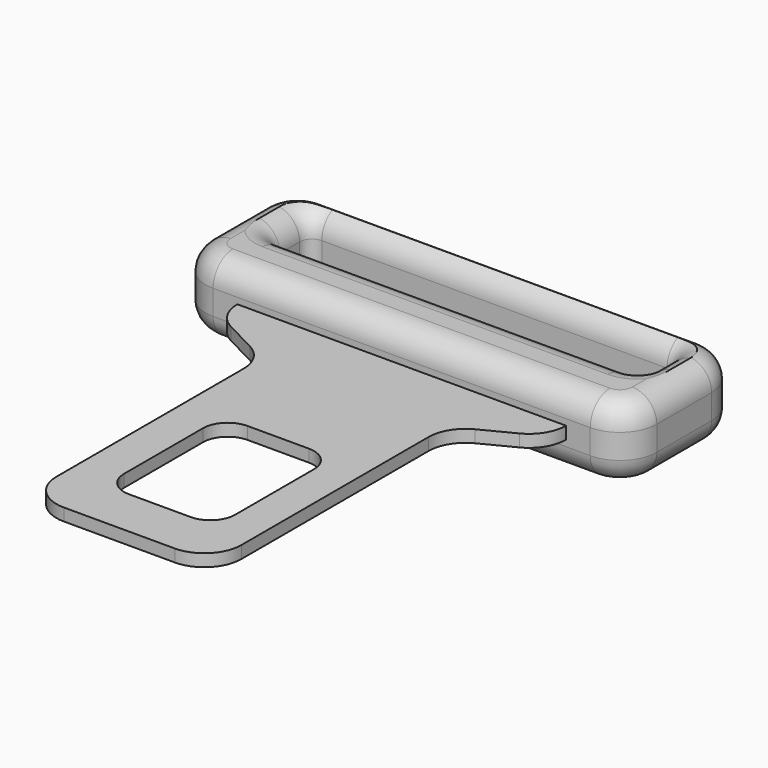
from build123d import *

# Parameters (mm, degrees)
F1_DEPTH     = 0.5
F2_DEPTH     = 3
F3_T1_DEPTH  = 30.5823954344
F3_T3_DEPTH  = 28
F3_T5_DEPTH  = 2
F3_T7_DEPTH  = 5.5512716671
F3_T10_ANGLE = 90
F3_T12_ANGLE = 90
F3_T14_ANGLE = 90
F3_T16_ANGLE = 90
F3_T18_ANGLE = 90
F3_T20_ANGLE = 90
F3_T22_ANGLE = 90
F3_T24_ANGLE = 90
F3_T26_ANGLE = 90
F3_T28_ANGLE = 90
F3_T30_ANGLE = 90
F3_T32_ANGLE = 90
F3_T34_ANGLE = 90
F3_T36_ANGLE = 90
F3_T38_ANGLE = 90
F3_T40_ANGLE = 90


# Not quite as in the source:
# - a fillet or chamfer that OpenCascade refuses, or shapes differently, is made with other operations: its cross-section is extruded or revolved along the edge and cut away or added
# - ends of sketch curves that miss each other by under 0.0002 mm in the source are joined


with BuildPart() as f1:
    # F0 (on Top) → F1 (new body, symmetric)
    with BuildSketch(Plane.XY):
        with BuildLine():
            ThreePointArc((-7.5000009313, -20.8021384721), (-6.6213212749, -22.9234588157), (-4.5000009313, -23.8021384721))
            Line((-4.5000009313, -23.8021384721), (4.4999990687, -23.8021384721))
            ThreePointArc((4.4999990687, -23.8021384721), (6.6213194122, -22.9234588157), (7.4999990687, -20.8021384721))
            Line((7.4999990687, -20.8021384721), (7.4999990687, -3.8021384721))
            Line((7.4999990687, -3.8021384721), (7.4999990687, -1.8323950848))
            ThreePointArc((7.4999990687, -1.8323950848), (7.9397973668, -0.2686280799), (9.1302438991, 0.8366442134))
            Line((9.1302438991, 0.8366442134), (11.6938184408, 2.1522747039))
            ThreePointArc((11.6938184408, 2.1522747039), (12.8842649732, 3.2575469972), (13.3240632713, 4.8213140021))
            Line((13.3240632713, 4.8213140021), (0, 4.8213140021))
            Line((0, 4.8213140021), (-13.3240632713, 4.8213140021))
            ThreePointArc((-13.3240632713, 4.8213140021), (-12.8842649732, 3.2575469972), (-11.6938184408, 2.1522747039))
            Line((-11.6938184408, 2.1522747039), (-9.1302438991, 0.8366442134))
            ThreePointArc((-9.1302438991, 0.8366442134), (-7.9397973668, -0.2686280799), (-7.4999990687, -1.8323950848))
            Line((-7.4999990687, -1.8323950848), (-7.4999990687, -3.8021384721))
            Line((-7.4999990687, -3.8021384721), (-7.5000009313, -20.8021384721))
        make_face()
        with BuildLine():
            ThreePointArc((-4.4058463536, -9.8073738366), (-3.820059916, -8.3931602743), (-2.4058463536, -7.8073738366))
            Line((-2.4058463536, -7.8073738366), (2.5941536464, -7.8073738366))
            ThreePointArc((2.5941536464, -7.8073738366), (4.0083672088, -8.3931602743), (4.5941536464, -9.8073738366))
            Line((4.5941536464, -9.8073738366), (4.5941536464, -17.8073738366))
            ThreePointArc((4.5941536464, -17.8073738366), (4.0083672088, -19.221587399), (2.5941536464, -19.8073738366))
            Line((2.5941536464, -19.8073738366), (-2.4058463536, -19.8073738366))
            ThreePointArc((-2.4058463536, -19.8073738366), (-3.820059916, -19.221587399), (-4.4058463536, -17.8073738366))
            Line((-4.4058463536, -17.8073738366), (-4.4058463536, -9.8073738366))
        make_face(mode=Mode.SUBTRACT)
    extrude(amount=F1_DEPTH, both=True)


with BuildPart() as f2:
    # F0 (on Top) → F2 (new body, symmetric)
    with BuildSketch(Plane.XY):
        with BuildLine():
            Line((-15.2911977172, 4.8213140021), (-13.3240632713, 4.8213140021))
            Line((-13.3240632713, 4.8213140021), (0, 4.8213140021))
            Line((0, 4.8213140021), (0, 10.225163497))
            Line((0, 10.225163497), (-14, 10.225163497))
            ThreePointArc((-14, 10.225163497), (-14.7071067812, 10.5180567158), (-15, 11.225163497))
            Line((-15, 11.225163497), (-15, 13.225163497))
            ThreePointArc((-15, 13.225163497), (-14.7071067812, 13.9322702782), (-14, 14.225163497))
            Line((-14, 14.225163497), (0, 14.225163497))
            Line((0, 14.225163497), (0, 16.3725856692))
            Line((0, 16.3725856692), (-15.2911977172, 16.3725856692))
            ThreePointArc((-15.2911977172, 16.3725856692), (-17.4125180607, 15.4939060127), (-18.2911977172, 13.3725856692))
            Line((-18.2911977172, 13.3725856692), (-18.2911977172, 7.8213140021))
            ThreePointArc((-18.2911977172, 7.8213140021), (-17.4125180607, 5.6999936585), (-15.2911977172, 4.8213140021))
        make_face()
        with BuildLine():
            Line((0, 4.8213140021), (13.3240632713, 4.8213140021))
            Line((13.3240632713, 4.8213140021), (15.2911977172, 4.8213140021))
            ThreePointArc((15.2911977172, 4.8213140021), (17.4125180607, 5.6999936585), (18.2911977172, 7.8213140021))
            Line((18.2911977172, 7.8213140021), (18.2911977172, 13.3725856692))
            ThreePointArc((18.2911977172, 13.3725856692), (17.4125180607, 15.4939060127), (15.2911977172, 16.3725856692))
            Line((15.2911977172, 16.3725856692), (0, 16.3725856692))
            Line((0, 16.3725856692), (0, 14.225163497))
            Line((0, 14.225163497), (14, 14.225163497))
            ThreePointArc((14, 14.225163497), (14.7071067812, 13.9322702782), (15, 13.225163497))
            Line((15, 13.225163497), (15, 11.225163497))
            ThreePointArc((15, 11.225163497), (14.7071067812, 10.5180567158), (14, 10.225163497))
            Line((14, 10.225163497), (0, 10.225163497))
            Line((0, 10.225163497), (0, 4.8213140021))
        make_face()
    extrude(amount=F2_DEPTH, both=True)

    # F3: fillet of radius 2 on 4 edges, made by hand

    # F3_s2 → F3_t1 (cut)
    with BuildSketch(Plane.YZ.offset(-15.2911977172)):
        with BuildLine():
            ThreePointArc((4.8213140021, 1), (5.4071004397, 2.4142135624), (6.8213140021, 3))
            Line((6.8213140021, 3), (4.8213140021, 3))
            Line((4.8213140021, 3), (4.8213140021, 1))
        make_face()
        with BuildLine():
            ThreePointArc((4.8213140021, -1), (5.4071004397, -2.4142135624), (6.8213140021, -3))
            Line((6.8213140021, -3), (4.8213140021, -3))
            Line((4.8213140021, -3), (4.8213140021, -1))
        make_face()
        with BuildLine():
            ThreePointArc((16.3725856692, -1), (15.7867992315, -2.4142135624), (14.3725856692, -3))
            Line((14.3725856692, -3), (16.3725856692, -3))
            Line((16.3725856692, -3), (16.3725856692, -1))
        make_face()
        with BuildLine():
            ThreePointArc((16.3725856692, 1), (15.7867992315, 2.4142135624), (14.3725856692, 3))
            Line((14.3725856692, 3), (16.3725856692, 3))
            Line((16.3725856692, 3), (16.3725856692, 1))
        make_face()
    extrude(amount=F3_T1_DEPTH, mode=Mode.SUBTRACT)

    # F3_s4 → F3_t3 (cut)
    with BuildSketch(Plane.YZ.offset(-14)):
        with BuildLine():
            ThreePointArc((16.225163497, 3), (14.8109499347, 2.4142135624), (14.225163497, 1))
            Line((14.225163497, 1), (14.225163497, 3))
            Line((14.225163497, 3), (16.225163497, 3))
        make_face()
        with BuildLine():
            ThreePointArc((14.225163497, -1), (14.8109499347, -2.4142135624), (16.225163497, -3))
            Line((16.225163497, -3), (14.225163497, -3))
            Line((14.225163497, -3), (14.225163497, -1))
        make_face()
        with BuildLine():
            ThreePointArc((10.225163497, -1), (9.6393770594, -2.4142135624), (8.225163497, -3))
            Line((8.225163497, -3), (10.225163497, -3))
            Line((10.225163497, -3), (10.225163497, -1))
        make_face()
        with BuildLine():
            ThreePointArc((8.225163497, 3), (9.6393770594, 2.4142135624), (10.225163497, 1))
            Line((10.225163497, 1), (10.225163497, 3))
            Line((10.225163497, 3), (8.225163497, 3))
        make_face()
    extrude(amount=F3_T3_DEPTH, mode=Mode.SUBTRACT)

    # F3_s6 → F3_t5 (cut)
    with BuildSketch(Plane.XZ.offset(-13.225163497)):
        with BuildLine():
            ThreePointArc((15, -1), (15.5857864376, -2.4142135624), (17, -3))
            Line((17, -3), (15, -3))
            Line((15, -3), (15, -1))
        make_face()
        with BuildLine():
            ThreePointArc((-15, -1), (-15.5857864376, -2.4142135624), (-17, -3))
            Line((-17, -3), (-15, -3))
            Line((-15, -3), (-15, -1))
        make_face()
        with BuildLine():
            ThreePointArc((17, 3), (15.5857864376, 2.4142135624), (15, 1))
            Line((15, 1), (15, 3))
            Line((15, 3), (17, 3))
        make_face()
        with BuildLine():
            ThreePointArc((-17, 3), (-15.5857864376, 2.4142135624), (-15, 1))
            Line((-15, 1), (-15, 3))
            Line((-15, 3), (-17, 3))
        make_face()
    extrude(amount=F3_T5_DEPTH, mode=Mode.SUBTRACT)

    # F3_s8 → F3_t7 (cut)
    with BuildSketch(Plane.XZ.offset(-13.3725856692)):
        with BuildLine():
            ThreePointArc((18.2911977172, -1), (17.7054112796, -2.4142135624), (16.2911977172, -3))
            Line((16.2911977172, -3), (18.2911977172, -3))
            Line((18.2911977172, -3), (18.2911977172, -1))
        make_face()
        with BuildLine():
            ThreePointArc((-18.2911977172, -1), (-17.7054112796, -2.4142135624), (-16.2911977172, -3))
            Line((-16.2911977172, -3), (-18.2911977172, -3))
            Line((-18.2911977172, -3), (-18.2911977172, -1))
        make_face()
        with BuildLine():
            ThreePointArc((18.2911977172, 1), (17.7054112796, 2.4142135624), (16.2911977172, 3))
            Line((16.2911977172, 3), (18.2911977172, 3))
            Line((18.2911977172, 3), (18.2911977172, 1))
        make_face()
        with BuildLine():
            ThreePointArc((-18.2911977172, 1), (-17.7054112796, 2.4142135624), (-16.2911977172, 3))
            Line((-16.2911977172, 3), (-18.2911977172, 3))
            Line((-18.2911977172, 3), (-18.2911977172, 1))
        make_face()
    extrude(amount=F3_T7_DEPTH, mode=Mode.SUBTRACT)

    # F3_s9 → F3_t10 (revolve, cut)
    with BuildSketch(Plane.XZ.offset(-13.225163497)):
        with BuildLine():
            ThreePointArc((-15, -1), (-15.5857864376, -2.4142135624), (-17, -3))
            Line((-17, -3), (-15, -3))
            Line((-15, -3), (-15, -1))
        make_face()
    revolve(axis=Axis((-14, 13.225163497, -3), (0, 0, -1)), revolution_arc=F3_T10_ANGLE, mode=Mode.SUBTRACT)

    # F3_s11 → F3_t12 (revolve, cut)
    with BuildSketch(Plane.YZ.offset(14)):
        with BuildLine():
            ThreePointArc((14.225163497, -1), (14.8109499347, -2.4142135624), (16.225163497, -3))
            Line((16.225163497, -3), (14.225163497, -3))
            Line((14.225163497, -3), (14.225163497, -1))
        make_face()
    revolve(axis=Axis((14, 13.225163497, -3), (0, 0, -1)), revolution_arc=F3_T12_ANGLE, mode=Mode.SUBTRACT)

    # F3_s13 → F3_t14 (revolve, cut)
    with BuildSketch(Plane.XZ.offset(-11.225163497)):
        with BuildLine():
            ThreePointArc((15, -1), (15.5857864376, -2.4142135624), (17, -3))
            Line((17, -3), (15, -3))
            Line((15, -3), (15, -1))
        make_face()
    revolve(axis=Axis((14, 11.225163497, -3), (0, 0, -1)), revolution_arc=F3_T14_ANGLE, mode=Mode.SUBTRACT)

    # F3_s15 → F3_t16 (revolve, cut)
    with BuildSketch(Plane.YZ.offset(-14)):
        with BuildLine():
            ThreePointArc((10.225163497, -1), (9.6393770594, -2.4142135624), (8.225163497, -3))
            Line((8.225163497, -3), (10.225163497, -3))
            Line((10.225163497, -3), (10.225163497, -1))
        make_face()
    revolve(axis=Axis((-14, 11.225163497, -3), (0, 0, -1)), revolution_arc=F3_T16_ANGLE, mode=Mode.SUBTRACT)

    # F3_s17 → F3_t18 (revolve, cut)
    with BuildSketch(Plane.XZ.offset(-13.225163497)):
        with BuildLine():
            ThreePointArc((-17, 3), (-15.5857864376, 2.4142135624), (-15, 1))
            Line((-15, 1), (-15, 3))
            Line((-15, 3), (-17, 3))
        make_face()
    revolve(axis=Axis((-14, 13.225163497, 3), (0, 0, -1)), revolution_arc=F3_T18_ANGLE, mode=Mode.SUBTRACT)

    # F3_s19 → F3_t20 (revolve, cut)
    with BuildSketch(Plane.YZ.offset(14)):
        with BuildLine():
            ThreePointArc((16.225163497, 3), (14.8109499347, 2.4142135624), (14.225163497, 1))
            Line((14.225163497, 1), (14.225163497, 3))
            Line((14.225163497, 3), (16.225163497, 3))
        make_face()
    revolve(axis=Axis((14, 13.225163497, 3), (0, 0, -1)), revolution_arc=F3_T20_ANGLE, mode=Mode.SUBTRACT)

    # F3_s21 → F3_t22 (revolve, cut)
    with BuildSketch(Plane.XZ.offset(-11.225163497)):
        with BuildLine():
            ThreePointArc((17, 3), (15.5857864376, 2.4142135624), (15, 1))
            Line((15, 1), (15, 3))
            Line((15, 3), (17, 3))
        make_face()
    revolve(axis=Axis((14, 11.225163497, 3), (0, 0, -1)), revolution_arc=F3_T22_ANGLE, mode=Mode.SUBTRACT)

    # F3_s23 → F3_t24 (revolve, cut)
    with BuildSketch(Plane.YZ.offset(-14)):
        with BuildLine():
            ThreePointArc((8.225163497, 3), (9.6393770594, 2.4142135624), (10.225163497, 1))
            Line((10.225163497, 1), (10.225163497, 3))
            Line((10.225163497, 3), (8.225163497, 3))
        make_face()
    revolve(axis=Axis((-14, 11.225163497, 3), (0, 0, -1)), revolution_arc=F3_T24_ANGLE, mode=Mode.SUBTRACT)

    # F3_s25 → F3_t26 (revolve, cut)
    with BuildSketch(Plane.XZ.offset(-7.8213140021)):
        with BuildLine():
            ThreePointArc((-18.2911977172, -1), (-17.7054112796, -2.4142135624), (-16.2911977172, -3))
            Line((-16.2911977172, -3), (-18.2911977172, -3))
            Line((-18.2911977172, -3), (-18.2911977172, -1))
        make_face()
    revolve(axis=Axis((-15.2911977172, 7.8213140021, -3), (0, 0, 1)), revolution_arc=F3_T26_ANGLE, mode=Mode.SUBTRACT)

    # F3_s27 → F3_t28 (revolve, cut)
    with BuildSketch(Plane.YZ.offset(15.2911977172)):
        with BuildLine():
            ThreePointArc((4.8213140021, -1), (5.4071004397, -2.4142135624), (6.8213140021, -3))
            Line((6.8213140021, -3), (4.8213140021, -3))
            Line((4.8213140021, -3), (4.8213140021, -1))
        make_face()
    revolve(axis=Axis((15.2911977172, 7.8213140021, -3), (0, 0, 1)), revolution_arc=F3_T28_ANGLE, mode=Mode.SUBTRACT)

    # F3_s29 → F3_t30 (revolve, cut)
    with BuildSketch(Plane.XZ.offset(-13.3725856692)):
        with BuildLine():
            ThreePointArc((18.2911977172, -1), (17.7054112796, -2.4142135624), (16.2911977172, -3))
            Line((16.2911977172, -3), (18.2911977172, -3))
            Line((18.2911977172, -3), (18.2911977172, -1))
        make_face()
    revolve(axis=Axis((15.2911977172, 13.3725856692, -3), (0, 0, 1)), revolution_arc=F3_T30_ANGLE, mode=Mode.SUBTRACT)

    # F3_s31 → F3_t32 (revolve, cut)
    with BuildSketch(Plane.YZ.offset(-15.2911977172)):
        with BuildLine():
            ThreePointArc((16.3725856692, -1), (15.7867992315, -2.4142135624), (14.3725856692, -3))
            Line((14.3725856692, -3), (16.3725856692, -3))
            Line((16.3725856692, -3), (16.3725856692, -1))
        make_face()
    revolve(axis=Axis((-15.2911977172, 13.3725856692, -3), (0, 0, 1)), revolution_arc=F3_T32_ANGLE, mode=Mode.SUBTRACT)

    # F3_s33 → F3_t34 (revolve, cut)
    with BuildSketch(Plane.XZ.offset(-7.8213140021)):
        with BuildLine():
            ThreePointArc((-18.2911977172, 1), (-17.7054112796, 2.4142135624), (-16.2911977172, 3))
            Line((-16.2911977172, 3), (-18.2911977172, 3))
            Line((-18.2911977172, 3), (-18.2911977172, 1))
        make_face()
    revolve(axis=Axis((-15.2911977172, 7.8213140021, 3), (0, 0, 1)), revolution_arc=F3_T34_ANGLE, mode=Mode.SUBTRACT)

    # F3_s35 → F3_t36 (revolve, cut)
    with BuildSketch(Plane.YZ.offset(15.2911977172)):
        with BuildLine():
            ThreePointArc((6.8213140021, 3), (5.4071004397, 2.4142135624), (4.8213140021, 1))
            Line((4.8213140021, 1), (4.8213140021, 3))
            Line((4.8213140021, 3), (6.8213140021, 3))
        make_face()
    revolve(axis=Axis((15.2911977172, 7.8213140021, 3), (0, 0, 1)), revolution_arc=F3_T36_ANGLE, mode=Mode.SUBTRACT)

    # F3_s37 → F3_t38 (revolve, cut)
    with BuildSketch(Plane.XZ.offset(-13.3725856692)):
        with BuildLine():
            ThreePointArc((18.2911977172, 1), (17.7054112796, 2.4142135624), (16.2911977172, 3))
            Line((16.2911977172, 3), (18.2911977172, 3))
            Line((18.2911977172, 3), (18.2911977172, 1))
        make_face()
    revolve(axis=Axis((15.2911977172, 13.3725856692, 3), (0, 0, 1)), revolution_arc=F3_T38_ANGLE, mode=Mode.SUBTRACT)

    # F3_s39 → F3_t40 (revolve, cut)
    with BuildSketch(Plane.YZ.offset(-15.2911977172)):
        with BuildLine():
            ThreePointArc((16.3725856692, 1), (15.7867992315, 2.4142135624), (14.3725856692, 3))
            Line((14.3725856692, 3), (16.3725856692, 3))
            Line((16.3725856692, 3), (16.3725856692, 1))
        make_face()
    revolve(axis=Axis((-15.2911977172, 13.3725856692, 3), (0, 0, 1)), revolution_arc=F3_T40_ANGLE, mode=Mode.SUBTRACT)


solid = Compound([f1.part, f2.part])
